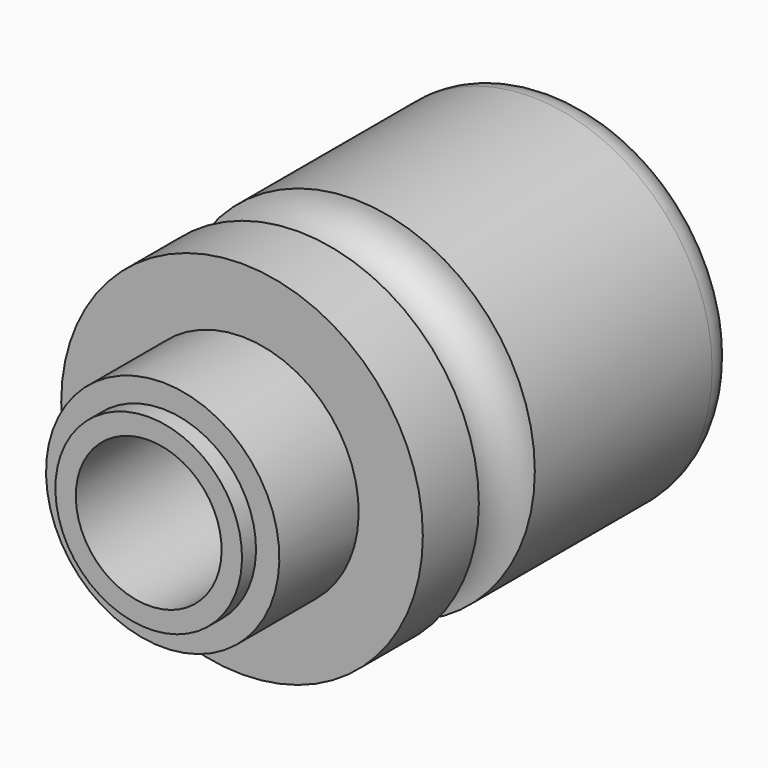
from build123d import *

# Parameters (mm, degrees)
F0_W = 3
F0_H = 3.5
F2_R = 5.99999


# Not quite as in the source:
# - a fillet or chamfer is up to 0.001 mm smaller than in the source, because OpenCascade refuses the exact size


with BuildPart() as f1:
    # F0 (on Right) → F1 (revolve)
    with BuildSketch(Plane.YZ):
        with Locations((-36.5, 14.25)):
            Rectangle(F0_W, F0_H)
        Polygon((-18, 12.5), (-18, 20), (-35, 20), (-35, 16), (-35, 12.5), align=None)
        Polygon((-6, 12.5), (-6, 31), (-18, 31), (-18, 20), (-18, 12.5), align=None)
        with BuildLine():
            Line((6, 12.5), (6, 31))
            ThreePointArc((6, 31), (0, 25), (-6, 31))
            Line((-6, 31), (-6, 12.5))
            Line((-6, 12.5), (6, 12.5))
        make_face()
        Polygon((50, 31), (6, 31), (6, 12.5), (20, 12.5), (20, 16), (28, 16), (28, 20.5), (35, 20.5), (35, 14), (38, 14), (38, 16), (48.5, 16), (48.5, 25), (50, 25), align=None)
    revolve(axis=Axis((0, 8.8457800448, 0), (0, 1, 0)))

    # F2 (radius 6 in the source; OpenCascade refuses exactly that, so slightly less here)
    f2_edges = [f1.edges().sort_by_distance(p)[0] for p in [
        (0, 50, -31),
    ]]
    fillet(f2_edges, radius=F2_R)


solid = f1.part
